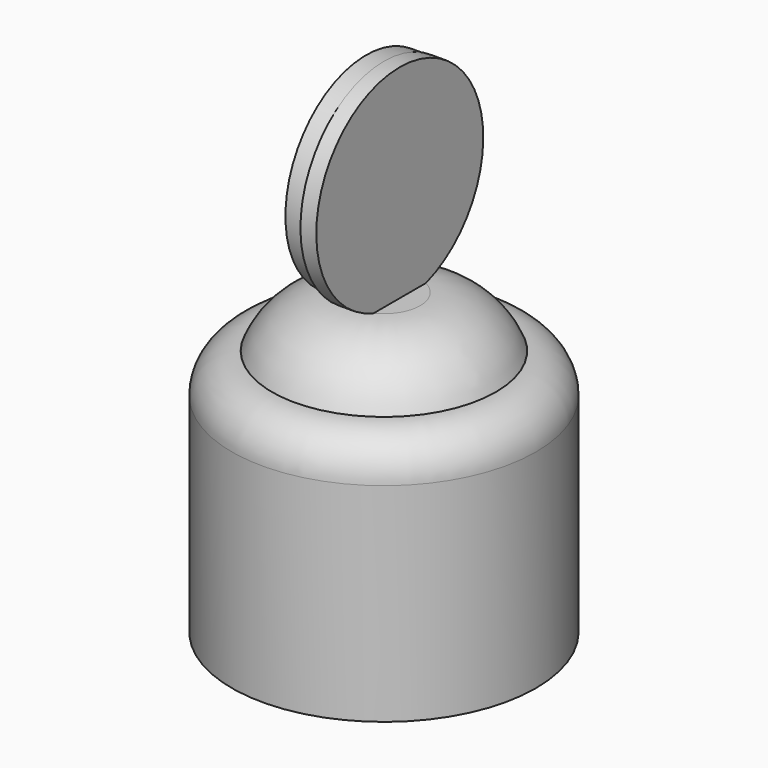
from build123d import *

# Parameters (mm, degrees)
F0_R     = 19.4994564254
F1_DEPTH = 31.75
F2_R     = 5.08
F3_R     = 14.3450562753
F4_DEPTH = 38.354
F6_R     = 13.3830864671
F7_DEPTH = 2.032
F8_R     = 12.9352143756
F9_DEPTH = 2.286


# Not quite as in the source:
# - a fillet or chamfer that OpenCascade refuses, or shapes differently, is made with other operations: its cross-section is extruded or revolved along the edge and cut away or added


with BuildPart() as f1:
    # F0 (on Top) → F1 (new body)
    with BuildSketch(Plane.XY):
        Circle(F0_R)
    extrude(amount=F1_DEPTH)

    # F2
    f2_edges = [f1.edges().sort_by_distance(p)[0] for p in [
        (-19.499456, 0, 31.75),
    ]]
    fillet(f2_edges, radius=F2_R)

    # F3 (on Top) → F4 (join)
    with BuildSketch(Plane.XY):
        Circle(F3_R)
    extrude(amount=F4_DEPTH)

    # F5: fillet of radius 10.4245741623 on 1 edges, made by hand

    # F5_s1 → F5_t2 (revolve, cut)
    with BuildSketch(Plane.XZ):
        with BuildLine():
            ThreePointArc((14.3450562753, 31.75), (10.5128533097, 36.5462583521), (4.6458315879, 38.354))
            Line((4.6458315879, 38.354), (14.3450562753, 38.354))
            Line((14.3450562753, 38.354), (14.3450562753, 31.75))
        make_face()
    revolve(axis=Axis((0, 0, 38.354), (0, 0, 1)), mode=Mode.SUBTRACT)

    # F6 (on Right) → F7 (join)
    with BuildSketch(Plane.YZ):
        with Locations((0, 51.0602071881)):
            Circle(F6_R)
    extrude(amount=F7_DEPTH)

    # F8 (on Right) → F9 (join)
    with BuildSketch(Plane.YZ):
        with Locations((0, 51.4653660357)):
            Circle(F8_R)
    extrude(amount=-F9_DEPTH)


solid = f1.part
